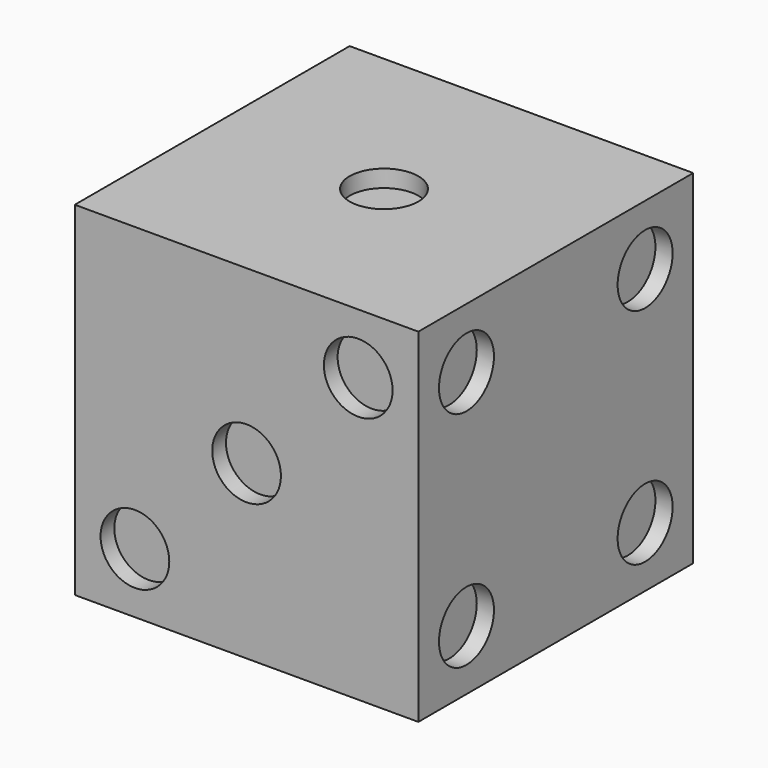
from build123d import *

# Parameters (mm, degrees)
F0_W      = 127
F0_H      = 127
F1_DEPTH  = 127
F2_R      = 12.7
F3_DEPTH  = 6.35
F4_R      = 12.7
F5_DEPTH  = 6.35
F6_R      = 12.7
F7_DEPTH  = 6.35
F8_R      = 12.7
F9_DEPTH  = 6.35
F10_R     = 12.7
F11_DEPTH = 6.35
F12_R     = 12.7
F13_DEPTH = 6.35


# Not quite as in the source:
# - a feature names something its author has since deleted; it is built from what else it names


with BuildPart() as f1:
    # F0 (on Top) → F1 (new body)
    with BuildSketch(Plane.XY):
        with Locations((63.5, 63.5)):
            Rectangle(F0_W, F0_H)
    extrude(amount=F1_DEPTH)

    # F2 (on face) → F3 (cut)
    with BuildSketch(Plane.XY.offset(127)):
        with Locations((63.5, 63.5)):
            Circle(F2_R)
    extrude(amount=-F3_DEPTH, mode=Mode.SUBTRACT)

    # F4 (on face) → F5 (cut)
    with BuildSketch(Plane(origin=(0, 0, 0), x_dir=(0, -1, 0), z_dir=(-1, 0, 0))):
        with Locations((-104.775, 22.225)):
            Circle(F4_R)
        with Locations((-22.225, 104.775)):
            Circle(F4_R)
    extrude(amount=-F5_DEPTH, mode=Mode.SUBTRACT)

    # F6 (on face) → F7 (cut)
    with BuildSketch(Plane.XZ):
        with Locations((22.225, 22.225)):
            Circle(F6_R)
        with Locations((63.5, 63.5)):
            Circle(F6_R)
        with Locations((104.775, 104.775)):
            Circle(F6_R)
    extrude(amount=-F7_DEPTH, mode=Mode.SUBTRACT)

    # F8 (on face) → F9 (cut)
    with BuildSketch(Plane.YZ.offset(127)):
        with Locations((22.225, 22.225)):
            Circle(F8_R)
        with Locations((22.225, 104.775)):
            Circle(F8_R)
        with Locations((104.775, 104.775)):
            Circle(F8_R)
        with Locations((104.775, 22.225)):
            Circle(F8_R)
    extrude(amount=-F9_DEPTH, mode=Mode.SUBTRACT)

    # F10 (on face) → F11 (cut)
    with BuildSketch(Plane(origin=(0, 127, 0), x_dir=(-1, 0, 0), z_dir=(0, 1, 0))):
        with Locations((-22.225, 22.225)):
            Circle(F10_R)
        with Locations((-104.775, 22.225)):
            Circle(F10_R)
        with Locations((-104.775, 104.775)):
            Circle(F10_R)
        with Locations((-22.225, 104.775)):
            Circle(F10_R)
        with Locations((-63.5, 63.5)):
            Circle(F10_R)
    extrude(amount=-F11_DEPTH, mode=Mode.SUBTRACT)

    # F12 (on face) → F13 (cut)
    with BuildSketch(Plane(origin=(0, 0, 0), x_dir=(1, 0, 0), z_dir=(0, 0, -1))):
        with Locations((22.225, -104.775)):
            Circle(F12_R)
        with Locations((104.775, -22.225)):
            Circle(F12_R)
        with Locations((22.225, -63.5)):
            Circle(F12_R)
        with Locations((104.775, -63.5)):
            Circle(F12_R)
        with Locations((104.775, -104.775)):
            Circle(F12_R)
        with Locations((22.225, -22.225)):
            Circle(F12_R)
    extrude(amount=-F13_DEPTH, mode=Mode.SUBTRACT)


solid = f1.part
